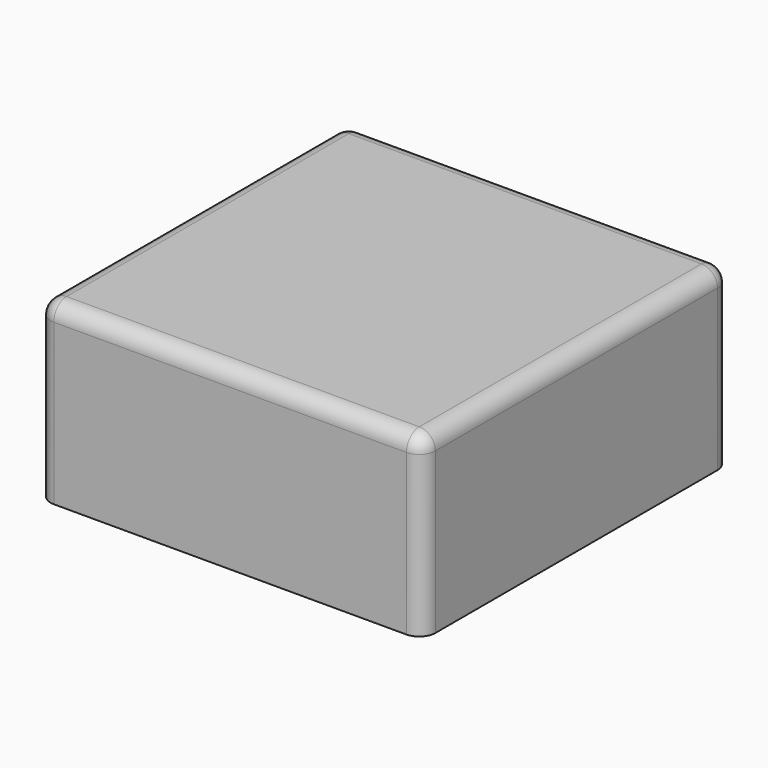
from build123d import *

# Parameters (mm, degrees)
F0_W     = 12
F0_H     = 12
F1_DEPTH = 5.5
F2_T     = -1
F3_W     = 1
F3_H     = 3
F4_DEPTH = 4.5
F6_W     = 1.3
F6_H     = 1.2
F6_W_2   = 1.2
F6_H_2   = 1.3
F7_DEPTH = 1.4
F8_R     = 0.5


with BuildPart() as f1:
    # F0 (on Top) → F1 (new body)
    with BuildSketch(Plane.XY):
        Rectangle(F0_W, F0_H)
    extrude(amount=F1_DEPTH)

    # F2
    f2_openings = [f1.faces().sort_by_distance(p)[0] for p in [
        (0, 0, 0),
    ]]
    offset(amount=F2_T, openings=f2_openings)

    # F3 (on face) → F4 (join, through all)
    with BuildSketch(Plane(origin=(0, 0, 4.5), x_dir=(1, 0, 0), z_dir=(0, 0, -1))):
        with Locations((2.4, 0.1532564508)):
            Rectangle(F3_W, F3_H)
        Polygon((0.6, 2.9), (0.6, 5), (0, 5), (-0.6, 5), (-0.6, 2.9), (-1.4, 2.9), (-1.4, 1.9), (0, 1.9), (1.4, 1.9), (1.4, 2.9), align=None)
        with Locations((-2.4, 0.1532564508)):
            Rectangle(F3_W, F3_H)
        Polygon((0, -1.9), (-1.4, -1.9), (-1.4, -2.9), (-0.6, -2.9), (-0.6, -5), (0, -5), (0.6, -5), (0.6, -2.9), (1.4, -2.9), (1.4, -1.9), align=None)
    extrude(amount=F4_DEPTH)

    # F6 (on face) → F7 (join, through all)
    with BuildSketch(Plane(origin=(0, 0, 4.5), x_dir=(1, 0, 0), z_dir=(0, 0, -1))):
        with Locations((1.25, 0)):
            Rectangle(F6_W, F6_H)
        Rectangle(F6_W_2, F6_H)
        with Locations((0, 1.25)):
            Rectangle(F6_W_2, F6_H_2)
        with Locations((-1.25, 0)):
            Rectangle(F6_W, F6_H)
        with Locations((0, -1.25)):
            Rectangle(F6_W_2, F6_H_2)
    extrude(amount=F7_DEPTH)

    # F8
    f8_edges = [f1.edges().sort_by_distance(p)[0] for p in [
        (6, 0, 5.5),
        (0, 6, 5.5),
        (-6, 0, 5.5),
        (0, -6, 5.5),
        (-6, 6, 2.75),
        (-6, -6, 2.75),
        (6, -6, 2.75),
        (6, 6, 2.75),
    ]]
    fillet(f8_edges, radius=F8_R)


solid = f1.part
